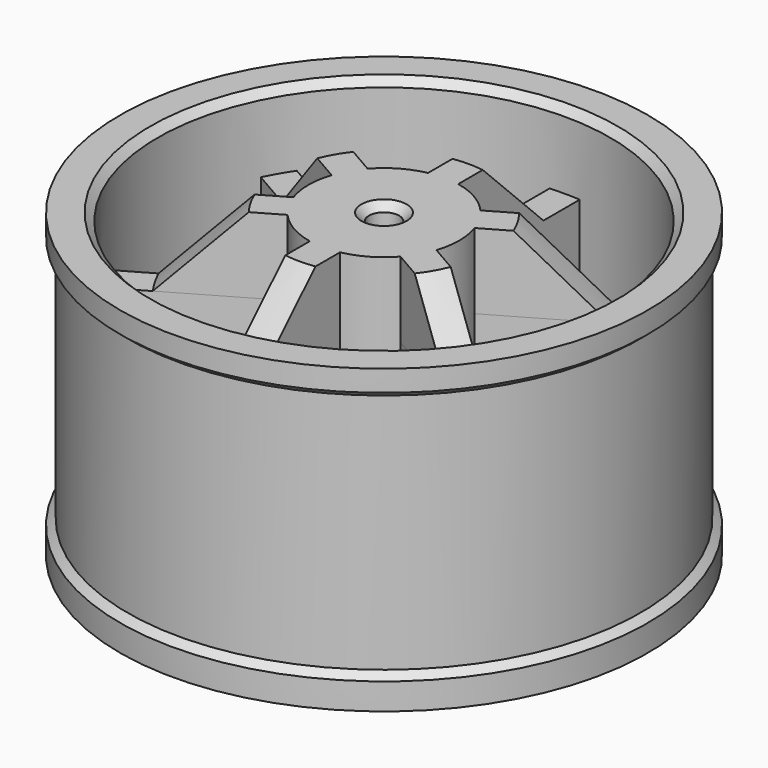
from build123d import *

# Parameters (mm, degrees)
F0_R          = 5
F0_R_2        = 1
F1_DEPTH      = 20
F0_R_3        = 17.5
F0_R_4        = 15
F2_W          = 2
F2_H          = 12
F3_DEPTH      = 15
F4_COUNT      = 6
F6_T4_ANGLE   = 359.64
F6_T11_ANGLE  = 359.64
F6_T18_ANGLE  = 359.64
F6_T25_ANGLE  = 359.64
F6_T32_ANGLE  = 359.64
F6_T39_ANGLE  = 359.64
F6_T46_ANGLE  = 359.64
F6_T53_ANGLE  = 359.64
F6_T60_ANGLE  = 359.64
F6_T67_ANGLE  = 359.64
F6_T74_ANGLE  = 359.64
F6_T81_ANGLE  = 359.64
F6_T88_ANGLE  = 359.64
F6_T95_ANGLE  = 359.64
F6_T102_ANGLE = 359.64
F6_T109_ANGLE = 359.64
F6_T116_ANGLE = 359.64
F6_T123_ANGLE = 359.64
F9_SIZE       = 0.5
F10_R         = 7
F10_R_2       = 3.5
F11_DEPTH     = 1.5
F12_SIZE      = 0.5


# Not quite as in the source:
# - a fillet or chamfer that OpenCascade refuses, or shapes differently, is made with other operations: its cross-section is extruded or revolved along the edge and cut away or added


with BuildPart() as f1:
    # F0 (on Top) → F1 (new body)
    with BuildSketch(Plane.XY):
        Circle(F0_R)
        Circle(F0_R_2, mode=Mode.SUBTRACT)
    extrude(amount=F1_DEPTH)



with BuildPart() as f1b:
    # F0 (on Top) → F1, piece 2 (new body)
    with BuildSketch(Plane.XY):
        Circle(F0_R_3)
        Circle(F0_R_4, mode=Mode.SUBTRACT)
    extrude(amount=F1_DEPTH)


with BuildPart() as f1_1:
    add(f1.part)

    add(f1b.part)  # F3 merges F1b
    # F2 (on Top) → F3 (join)
    with BuildSketch(Plane.XY):
        with Locations((0, 10)):
            Rectangle(F2_W, F2_H)
    extrude(amount=F3_DEPTH)


with BuildPart() as f4_1:
    # F4: instance of F1
    add(f1_1.part.rotate(Axis((0, 0, 0), (0, 0, -1)), 1 * 360 / F4_COUNT))


with BuildPart() as f4_2:
    # F4: instance of F1
    add(f1_1.part.rotate(Axis((0, 0, 0), (0, 0, -1)), 2 * 360 / F4_COUNT))


with BuildPart() as f4_3:
    # F4: instance of F1
    add(f1_1.part.rotate(Axis((0, 0, 0), (0, 0, -1)), 3 * 360 / F4_COUNT))


with BuildPart() as f4_4:
    # F4: instance of F1
    add(f1_1.part.rotate(Axis((0, 0, 0), (0, 0, -1)), 4 * 360 / F4_COUNT))


with BuildPart() as f4_5:
    # F4: instance of F1
    add(f1_1.part.rotate(Axis((0, 0, 0), (0, 0, -1)), 5 * 360 / F4_COUNT))


with BuildPart() as f4_4_1:
    add(f4_4.part)

    # F5: union F4_1, F4_2, F4_3, F1, F4_5
    add(f4_1.part)
    add(f4_2.part)
    add(f4_3.part)
    add(f1_1.part)
    add(f4_5.part)

    # F6: chamfer of 7 on 6 edges, made by hand


with BuildPart() as f6_tool2:
    # F6_s3 → F6_t4 (revolve)
    with BuildSketch(Plane(origin=(0, 0, 0), x_dir=(0, 0, 1), z_dir=(-0.5027182272, -0.8644503364, 0))):
        Polygon((22, 5), (15, 12), (15, 5), align=None)
    revolve(axis=Axis((0, 0, 15), (0, 0, -1)), revolution_arc=F6_T4_ANGLE)

    split(bisect_by=Plane(origin=(0.5, 0.8660254038, 0), x_dir=(0, 0, 1), z_dir=(-0.5, -0.8660254038, 0)), keep=Keep.TOP)

    split(bisect_by=Plane.XY.offset(20), keep=Keep.BOTTOM)

    split(bisect_by=Plane(origin=(-0.5, -0.8660254038, 0), x_dir=(0, 0, 1), z_dir=(0.5, 0.8660254038, 0)), keep=Keep.TOP)


with BuildPart() as f4_4_2:
    add(f4_4_1.part)

    # F6_t1: union F6_tool2
    add(f6_tool2.part)


with BuildPart() as f6_tool9:
    # F6_s10 → F6_t11 (revolve)
    with BuildSketch(Plane(origin=(0, 0, 0), x_dir=(0, 0, 1), z_dir=(-0.5027182272, -0.8644503364, 0))):
        Polygon((22, 5), (15, 12), (15, 5), align=None)
    revolve(axis=Axis((0, 0, 15), (0, 0, -1)), revolution_arc=F6_T11_ANGLE)

    split(bisect_by=Plane.XY.offset(20), keep=Keep.BOTTOM)

    split(bisect_by=Plane.YZ.offset(-1), keep=Keep.TOP)

    split(bisect_by=Plane.YZ.offset(1), keep=Keep.BOTTOM)


with BuildPart() as f4_4_3:
    add(f4_4_2.part)

    # F6_t8: union F6_tool9
    add(f6_tool9.part)


with BuildPart() as f6_tool16:
    # F6_s17 → F6_t18 (revolve)
    with BuildSketch(Plane(origin=(0, 0, 0), x_dir=(0, 0, 1), z_dir=(-0.5027182272, -0.8644503364, 0))):
        Polygon((22, 5), (15, 12), (15, 5), align=None)
    revolve(axis=Axis((0, 0, 15), (0, 0, -1)), revolution_arc=F6_T18_ANGLE)

    split(bisect_by=Plane.XY.offset(20), keep=Keep.BOTTOM)

    split(bisect_by=Plane(origin=(-0.5, 0.8660254038, 0), x_dir=(0, 0, 1), z_dir=(0.5, -0.8660254038, 0)), keep=Keep.TOP)

    split(bisect_by=Plane(origin=(0.5, -0.8660254038, 0), x_dir=(0, 0, 1), z_dir=(-0.5, 0.8660254038, 0)), keep=Keep.TOP)


with BuildPart() as f4_4_4:
    add(f4_4_3.part)

    # F6_t15: union F6_tool16
    add(f6_tool16.part)


with BuildPart() as f6_tool23:
    # F6_s24 → F6_t25 (revolve)
    with BuildSketch(Plane(origin=(0, 0, 0), x_dir=(0, 0, 1), z_dir=(0.497276838, -0.8675919239, 0))):
        Polygon((22, 5), (15, 12), (15, 5), align=None)
    revolve(axis=Axis((0, 0, 15), (0, 0, -1)), revolution_arc=F6_T25_ANGLE)

    split(bisect_by=Plane.XY.offset(20), keep=Keep.BOTTOM)

    split(bisect_by=Plane(origin=(-0.5, 0.8660254038, 0), x_dir=(0, 0, 1), z_dir=(0.5, -0.8660254038, 0)), keep=Keep.TOP)

    split(bisect_by=Plane(origin=(0.5, -0.8660254038, 0), x_dir=(0, 0, 1), z_dir=(-0.5, 0.8660254038, 0)), keep=Keep.TOP)


with BuildPart() as f4_4_5:
    add(f4_4_4.part)

    # F6_t22: union F6_tool23
    add(f6_tool23.part)


with BuildPart() as f6_tool30:
    # F6_s31 → F6_t32 (revolve)
    with BuildSketch(Plane(origin=(0, 0, 0), x_dir=(0, 0, 1), z_dir=(0.497276838, -0.8675919239, 0))):
        Polygon((22, 5), (15, 12), (15, 5), align=None)
    revolve(axis=Axis((0, 0, 15), (0, 0, -1)), revolution_arc=F6_T32_ANGLE)

    split(bisect_by=Plane(origin=(0.5, 0.8660254038, 0), x_dir=(0, 0, 1), z_dir=(-0.5, -0.8660254038, 0)), keep=Keep.TOP)

    split(bisect_by=Plane.XY.offset(20), keep=Keep.BOTTOM)

    split(bisect_by=Plane(origin=(-0.5, -0.8660254038, 0), x_dir=(0, 0, 1), z_dir=(0.5, 0.8660254038, 0)), keep=Keep.TOP)


with BuildPart() as f4_4_6:
    add(f4_4_5.part)

    # F6_t29: union F6_tool30
    add(f6_tool30.part)


with BuildPart() as f6_tool37:
    # F6_s38 → F6_t39 (revolve)
    with BuildSketch(Plane(origin=(0, 0, 0), x_dir=(0, 0, 1), z_dir=(0.497276838, -0.8675919239, 0))):
        Polygon((22, 5), (15, 12), (15, 5), align=None)
    revolve(axis=Axis((0, 0, 15), (0, 0, -1)), revolution_arc=F6_T39_ANGLE)

    split(bisect_by=Plane.XY.offset(20), keep=Keep.BOTTOM)

    split(bisect_by=Plane.YZ.offset(-1), keep=Keep.TOP)

    split(bisect_by=Plane.YZ.offset(1), keep=Keep.BOTTOM)


with BuildPart() as f4_4_7:
    add(f4_4_6.part)

    # F6_t36: union F6_tool37
    add(f6_tool37.part)


with BuildPart() as f6_tool44:
    # F6_s45 → F6_t46 (revolve)
    with BuildSketch(Plane(origin=(0, 0, 0), x_dir=(0, 0, 1), z_dir=(0.9999950652, -0.0031415875, 0))):
        Polygon((22, 5), (15, 12), (15, 5), align=None)
    revolve(axis=Axis((0, 0, 15), (0, 0, -1)), revolution_arc=F6_T46_ANGLE)

    split(bisect_by=Plane.XY.offset(20), keep=Keep.BOTTOM)

    split(bisect_by=Plane.YZ.offset(-1), keep=Keep.TOP)

    split(bisect_by=Plane.YZ.offset(1), keep=Keep.BOTTOM)


with BuildPart() as f4_4_8:
    add(f4_4_7.part)

    # F6_t43: union F6_tool44
    add(f6_tool44.part)


with BuildPart() as f6_tool51:
    # F6_s52 → F6_t53 (revolve)
    with BuildSketch(Plane(origin=(0, 0, 0), x_dir=(0, 0, 1), z_dir=(0.9999950652, -0.0031415875, 0))):
        Polygon((22, 5), (15, 12), (15, 5), align=None)
    revolve(axis=Axis((0, 0, 15), (0, 0, -1)), revolution_arc=F6_T53_ANGLE)

    split(bisect_by=Plane.XY.offset(20), keep=Keep.BOTTOM)

    split(bisect_by=Plane(origin=(-0.5, 0.8660254038, 0), x_dir=(0, 0, 1), z_dir=(0.5, -0.8660254038, 0)), keep=Keep.TOP)

    split(bisect_by=Plane(origin=(0.5, -0.8660254038, 0), x_dir=(0, 0, 1), z_dir=(-0.5, 0.8660254038, 0)), keep=Keep.TOP)


with BuildPart() as f4_4_9:
    add(f4_4_8.part)

    # F6_t50: union F6_tool51
    add(f6_tool51.part)


with BuildPart() as f6_tool58:
    # F6_s59 → F6_t60 (revolve)
    with BuildSketch(Plane(origin=(0, 0, 0), x_dir=(0, 0, 1), z_dir=(0.9999950652, -0.0031415875, 0))):
        Polygon((22, 5), (15, 12), (15, 5), align=None)
    revolve(axis=Axis((0, 0, 15), (0, 0, -1)), revolution_arc=F6_T60_ANGLE)

    split(bisect_by=Plane(origin=(0.5, 0.8660254038, 0), x_dir=(0, 0, 1), z_dir=(-0.5, -0.8660254038, 0)), keep=Keep.TOP)

    split(bisect_by=Plane.XY.offset(20), keep=Keep.BOTTOM)

    split(bisect_by=Plane(origin=(-0.5, -0.8660254038, 0), x_dir=(0, 0, 1), z_dir=(0.5, 0.8660254038, 0)), keep=Keep.TOP)


with BuildPart() as f4_4_10:
    add(f4_4_9.part)

    # F6_t57: union F6_tool58
    add(f6_tool58.part)


with BuildPart() as f6_tool65:
    # F6_s66 → F6_t67 (revolve)
    with BuildSketch(Plane(origin=(0, 0, 0), x_dir=(0, 0, 1), z_dir=(0.5027182272, 0.8644503364, 0))):
        Polygon((22, 5), (15, 12), (15, 5), align=None)
    revolve(axis=Axis((0, 0, 15), (0, 0, -1)), revolution_arc=F6_T67_ANGLE)

    split(bisect_by=Plane(origin=(0.5, 0.8660254038, 0), x_dir=(0, 0, 1), z_dir=(-0.5, -0.8660254038, 0)), keep=Keep.TOP)

    split(bisect_by=Plane.XY.offset(20), keep=Keep.BOTTOM)

    split(bisect_by=Plane(origin=(-0.5, -0.8660254038, 0), x_dir=(0, 0, 1), z_dir=(0.5, 0.8660254038, 0)), keep=Keep.TOP)


with BuildPart() as f4_4_11:
    add(f4_4_10.part)

    # F6_t64: union F6_tool65
    add(f6_tool65.part)


with BuildPart() as f6_tool72:
    # F6_s73 → F6_t74 (revolve)
    with BuildSketch(Plane(origin=(0, 0, 0), x_dir=(0, 0, 1), z_dir=(0.5027182272, 0.8644503364, 0))):
        Polygon((22, 5), (15, 12), (15, 5), align=None)
    revolve(axis=Axis((0, 0, 15), (0, 0, -1)), revolution_arc=F6_T74_ANGLE)

    split(bisect_by=Plane.XY.offset(20), keep=Keep.BOTTOM)

    split(bisect_by=Plane.YZ.offset(-1), keep=Keep.TOP)

    split(bisect_by=Plane.YZ.offset(1), keep=Keep.BOTTOM)


with BuildPart() as f4_4_12:
    add(f4_4_11.part)

    # F6_t71: union F6_tool72
    add(f6_tool72.part)


with BuildPart() as f6_tool79:
    # F6_s80 → F6_t81 (revolve)
    with BuildSketch(Plane(origin=(0, 0, 0), x_dir=(0, 0, 1), z_dir=(0.5027182272, 0.8644503364, 0))):
        Polygon((22, 5), (15, 12), (15, 5), align=None)
    revolve(axis=Axis((0, 0, 15), (0, 0, -1)), revolution_arc=F6_T81_ANGLE)

    split(bisect_by=Plane.XY.offset(20), keep=Keep.BOTTOM)

    split(bisect_by=Plane(origin=(-0.5, 0.8660254038, 0), x_dir=(0, 0, 1), z_dir=(0.5, -0.8660254038, 0)), keep=Keep.TOP)

    split(bisect_by=Plane(origin=(0.5, -0.8660254038, 0), x_dir=(0, 0, 1), z_dir=(-0.5, 0.8660254038, 0)), keep=Keep.TOP)


with BuildPart() as f4_4_13:
    add(f4_4_12.part)

    # F6_t78: union F6_tool79
    add(f6_tool79.part)


with BuildPart() as f6_tool86:
    # F6_s87 → F6_t88 (revolve)
    with BuildSketch(Plane(origin=(0, 0, 0), x_dir=(0, 0, 1), z_dir=(-0.497276838, 0.8675919239, 0))):
        Polygon((22, 5), (15, 12), (15, 5), align=None)
    revolve(axis=Axis((0, 0, 15), (0, 0, -1)), revolution_arc=F6_T88_ANGLE)

    split(bisect_by=Plane.XY.offset(20), keep=Keep.BOTTOM)

    split(bisect_by=Plane(origin=(-0.5, 0.8660254038, 0), x_dir=(0, 0, 1), z_dir=(0.5, -0.8660254038, 0)), keep=Keep.TOP)

    split(bisect_by=Plane(origin=(0.5, -0.8660254038, 0), x_dir=(0, 0, 1), z_dir=(-0.5, 0.8660254038, 0)), keep=Keep.TOP)


with BuildPart() as f4_4_14:
    add(f4_4_13.part)

    # F6_t85: union F6_tool86
    add(f6_tool86.part)


with BuildPart() as f6_tool93:
    # F6_s94 → F6_t95 (revolve)
    with BuildSketch(Plane(origin=(0, 0, 0), x_dir=(0, 0, 1), z_dir=(-0.497276838, 0.8675919239, 0))):
        Polygon((22, 5), (15, 12), (15, 5), align=None)
    revolve(axis=Axis((0, 0, 15), (0, 0, -1)), revolution_arc=F6_T95_ANGLE)

    split(bisect_by=Plane(origin=(0.5, 0.8660254038, 0), x_dir=(0, 0, 1), z_dir=(-0.5, -0.8660254038, 0)), keep=Keep.TOP)

    split(bisect_by=Plane.XY.offset(20), keep=Keep.BOTTOM)

    split(bisect_by=Plane(origin=(-0.5, -0.8660254038, 0), x_dir=(0, 0, 1), z_dir=(0.5, 0.8660254038, 0)), keep=Keep.TOP)


with BuildPart() as f4_4_15:
    add(f4_4_14.part)

    # F6_t92: union F6_tool93
    add(f6_tool93.part)


with BuildPart() as f6_tool100:
    # F6_s101 → F6_t102 (revolve)
    with BuildSketch(Plane(origin=(0, 0, 0), x_dir=(0, 0, 1), z_dir=(-0.497276838, 0.8675919239, 0))):
        Polygon((22, 5), (15, 12), (15, 5), align=None)
    revolve(axis=Axis((0, 0, 15), (0, 0, -1)), revolution_arc=F6_T102_ANGLE)

    split(bisect_by=Plane.XY.offset(20), keep=Keep.BOTTOM)

    split(bisect_by=Plane.YZ.offset(-1), keep=Keep.TOP)

    split(bisect_by=Plane.YZ.offset(1), keep=Keep.BOTTOM)


with BuildPart() as f4_4_16:
    add(f4_4_15.part)

    # F6_t99: union F6_tool100
    add(f6_tool100.part)


with BuildPart() as f6_tool107:
    # F6_s108 → F6_t109 (revolve)
    with BuildSketch(Plane(origin=(0, 0, 0), x_dir=(0, 0, 1), z_dir=(-0.9999950652, 0.0031415875, 0))):
        Polygon((22, 5), (15, 12), (15, 5), align=None)
    revolve(axis=Axis((0, 0, 15), (0, 0, -1)), revolution_arc=F6_T109_ANGLE)

    split(bisect_by=Plane.XY.offset(20), keep=Keep.BOTTOM)

    split(bisect_by=Plane.YZ.offset(-1), keep=Keep.TOP)

    split(bisect_by=Plane.YZ.offset(1), keep=Keep.BOTTOM)


with BuildPart() as f4_4_17:
    add(f4_4_16.part)

    # F6_t106: union F6_tool107
    add(f6_tool107.part)


with BuildPart() as f6_tool114:
    # F6_s115 → F6_t116 (revolve)
    with BuildSketch(Plane(origin=(0, 0, 0), x_dir=(0, 0, 1), z_dir=(-0.9999950652, 0.0031415875, 0))):
        Polygon((22, 5), (15, 12), (15, 5), align=None)
    revolve(axis=Axis((0, 0, 15), (0, 0, -1)), revolution_arc=F6_T116_ANGLE)

    split(bisect_by=Plane.XY.offset(20), keep=Keep.BOTTOM)

    split(bisect_by=Plane(origin=(-0.5, 0.8660254038, 0), x_dir=(0, 0, 1), z_dir=(0.5, -0.8660254038, 0)), keep=Keep.TOP)

    split(bisect_by=Plane(origin=(0.5, -0.8660254038, 0), x_dir=(0, 0, 1), z_dir=(-0.5, 0.8660254038, 0)), keep=Keep.TOP)


with BuildPart() as f4_4_18:
    add(f4_4_17.part)

    # F6_t113: union F6_tool114
    add(f6_tool114.part)


with BuildPart() as f6_tool121:
    # F6_s122 → F6_t123 (revolve)
    with BuildSketch(Plane(origin=(0, 0, 0), x_dir=(0, 0, 1), z_dir=(-0.9999950652, 0.0031415875, 0))):
        Polygon((22, 5), (15, 12), (15, 5), align=None)
    revolve(axis=Axis((0, 0, 15), (0, 0, -1)), revolution_arc=F6_T123_ANGLE)

    split(bisect_by=Plane(origin=(0.5, 0.8660254038, 0), x_dir=(0, 0, 1), z_dir=(-0.5, -0.8660254038, 0)), keep=Keep.TOP)

    split(bisect_by=Plane.XY.offset(20), keep=Keep.BOTTOM)

    split(bisect_by=Plane(origin=(-0.5, -0.8660254038, 0), x_dir=(0, 0, 1), z_dir=(0.5, 0.8660254038, 0)), keep=Keep.TOP)


with BuildPart() as f4_4_19:
    add(f4_4_18.part)

    # F6_t120: union F6_tool121
    add(f6_tool121.part)

    # F7 (on Front) → F8 (revolve, cut)
    with BuildSketch(Plane.XZ):
        Polygon((-17, 18.1724479471), (-20.0641777725, 20.7435983859), (-20.0641777725, -0.3987024916), (-17, 2.1724479471), align=None)
    revolve(axis=Axis((0, 0, 20), (0, 0, 1)), mode=Mode.SUBTRACT)

    # F9
    f9_edges = [f4_4_19.edges().sort_by_distance(p)[0] for p in [
        (0.5, -0.866025, 20),
        (7.5, -12.990381, 20),
    ]]
    chamfer(f9_edges, length=F9_SIZE)

    # F10 (on face) → F11 (join)
    with BuildSketch(Plane(origin=(0, 0, 0), x_dir=(1, 0, 0), z_dir=(0, 0, -1))):
        Circle(F10_R)
        Circle(F10_R_2, mode=Mode.SUBTRACT)
        with BuildLine():
            ThreePointArc((1, -6.9282032303), (3.5, -6.0621778265), (5.5, -4.3301270189))
            Line((5.5, -4.3301270189), (3.7426406871, -3.3155151466))
            ThreePointArc((3.7426406871, -3.3155151466), (2.5, -4.3301270189), (1, -4.8989794856))
            Line((1, -4.8989794856), (1, -6.9282032303))
        make_face()
    extrude(amount=-F11_DEPTH)

    # F12
    f12_edges = [f4_4_19.edges().sort_by_distance(p)[0] for p in [
        (0.5, -0.866025, 0),
    ]]
    chamfer(f12_edges, length=F12_SIZE)


solid = f4_4_19.part
